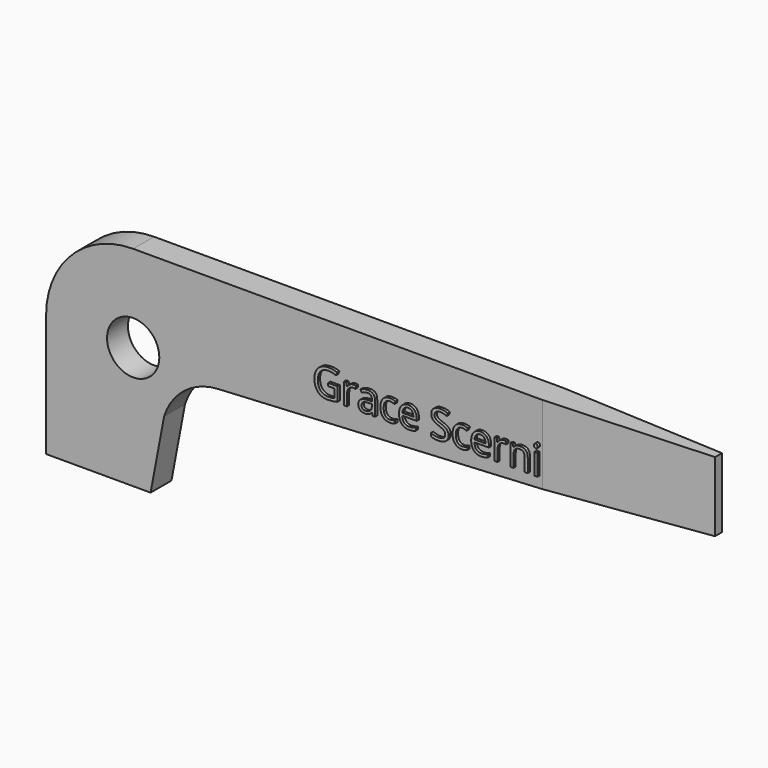
from build123d import *

# Parameters (mm, degrees)
F1_DEPTH     = 2.38125
F2_R         = 2.38125
F3_DEPTH     = 2.38225
F5_DEPTH     = 25.4
F6_TEXT_SIZE = 3.5641521096
F7_DEPTH     = 0.254


# Not quite as in the source:
# - Text() gives the source's letters only with a copy of the font that has no kerning and outlines rounded to 1/6400 em; it was checked with that copy


with BuildPart() as f1:
    # F0 (on Front) → F1 (new body)
    with BuildSketch(Plane.XZ):
        with BuildLine():
            Line((60.325, 19.05), (7.9375, 19.05))
            ThreePointArc((7.9375, 19.05), (2.3248399243, 16.7251600757), (0, 11.1125))
            Line((0, 11.1125), (0, 0))
            Line((0, 0), (9.525, 0))
            Line((9.525, 0), (10.7566304505, 6.52649533))
            ThreePointArc((10.7566304505, 6.52649533), (12.6183721925, 9.1883752642), (15.6634210502, 10.3194652484))
            Line((15.6634210502, 10.3194652484), (60.325, 12.7))
            Line((60.325, 12.7), (60.325, 19.05))
        make_face()
    extrude(amount=F1_DEPTH)

    # F2 (on face) → F3 (cut, through all)
    with BuildSketch(Plane.XZ.offset(2.38125)):
        with Locations((7.9375, 11.1125)):
            Circle(F2_R)
    extrude(amount=-F3_DEPTH, mode=Mode.SUBTRACT)

    # F4 (on face) → F5 (cut)
    with BuildSketch(Plane.XY.offset(19.05)):
        Polygon((60.325, -2.38125), (60.325, -1.5875), (45.24375, -2.38125), align=None)
        Polygon((45.24375, 0), (60.325, -0.79375), (60.325, 0), align=None)
    extrude(amount=-F5_DEPTH, mode=Mode.SUBTRACT)

    # F6 (on face) → F7 (join)
    with BuildSketch(Plane.XZ.offset(2.38125)):
        with Locations((24.4391258576, 12.9068829119)):
            Text('Grace Scerni', F6_TEXT_SIZE, font='Open Sans', text_align=(TextAlign.LEFT, TextAlign.BOTTOM))
    extrude(amount=F7_DEPTH)


solid = f1.part
